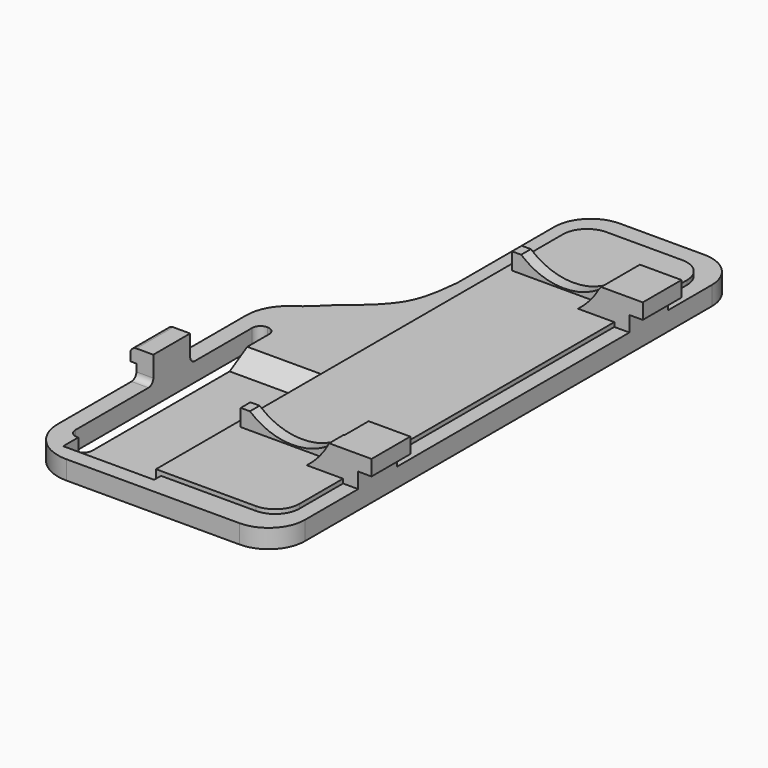
from build123d import *

# Parameters (mm, degrees)
F1_DEPTH     = 1.55
F3_DEPTH     = 0.35
F4_W         = 8.65
F4_H         = 1
F5_DEPTH     = 1.3
F7_W         = 4.25
F7_H         = 4
F8_DEPTH     = 2.55
F10_DEPTH    = 39.5010001
F11_W        = 4
F11_H        = 1.275
F12_DEPTH    = 1.1
F13_W        = 8.65
F13_H        = 1
F14_DEPTH    = 1.4
F15_DEPTH    = 38.0010001
F17_DEPTH    = 1.4
F18_T4_DEPTH = 11.4290603676
F19_T4_DEPTH = 10.6517870966
F20_W        = 1.4
F20_H        = 3.8
F21_DEPTH    = 2.2
F22_W        = 3.8
F22_H        = 1.1
F23_DEPTH    = 0.5
F24_R        = 0.5


# Not quite as in the source:
# - a fillet or chamfer that OpenCascade refuses, or shapes differently, is made with other operations: its cross-section is extruded or revolved along the edge and cut away or added


with BuildPart() as f1:
    # F0 (on Top) → F1 (new body)
    with BuildSketch(Plane.XY):
        with BuildLine():
            Line((-12.4797472133, -24.9172599055), (1.8202527867, -24.9172599055))
            ThreePointArc((1.8202527867, -24.9172599055), (3.9415731303, -24.038580249), (4.8202527867, -21.9172599055))
            Line((4.8202527867, -21.9172599055), (4.8202527867, 20.0827400945))
            ThreePointArc((4.8202527867, 20.0827400945), (3.9415731303, 22.2040604381), (1.8202527867, 23.0827400945))
            Line((1.8202527867, 23.0827400945), (-5.1797472133, 23.0827400945))
            ThreePointArc((-5.1797472133, 23.0827400945), (-7.3010675568, 22.2040604381), (-8.1797472133, 20.0827400945))
            Line((-8.1797472133, 20.0827400945), (-8.1797472133, 10.0827400945))
            add(Edge.make_bspline(
                [(-8.1797472133, 10.0827400945), (-8.4297074571, 7.300546721), (-9.1785947804, 5.6351239407), (-11.0454632546, 3.7753203501), (-12.7602456599, 2.4755173938), (-13.6481305175, 1.4367913649), (-14.42578763, 0.9165801451)],
                knots=[0, 0, 0, 0, 0.3064186573, 0.5153311453, 0.7233584291, 0.9057268673, 0.9057268673, 0.9057268673, 0.9057268673], degree=3))
            ThreePointArc((-14.42578763, 0.9165801451), (-15.5669094587, -0.3434616219), (-15.9797472133, -1.9925308353))
            Line((-15.9797472133, -1.9925308353), (-15.9797472133, -21.4172599055))
            ThreePointArc((-15.9797472133, -21.4172599055), (-14.9546209474, -23.8921336396), (-12.4797472133, -24.9172599055))
        make_face()
        with BuildLine():
            Line((-14.5797472133, -21.3672599055), (-14.5797472133, -3.1172599055))
            ThreePointArc((-14.5797472133, -3.1172599055), (-14.3747219601, -2.6222851587), (-13.8797472133, -2.4172599055))
            ThreePointArc((-13.8797472133, -2.4172599055), (-13.3847724664, -2.6222851587), (-13.1797472133, -3.1172599055))
            Line((-13.1797472133, -3.1172599055), (-13.1797472133, -21.3672599055))
            ThreePointArc((-13.1797472133, -21.3672599055), (-13.3847724664, -21.8622346523), (-13.8797472133, -22.0672599055))
            ThreePointArc((-13.8797472133, -22.0672599055), (-14.3747219601, -21.8622346523), (-14.5797472133, -21.3672599055))
        make_face(mode=Mode.SUBTRACT)
    extrude(amount=F1_DEPTH)

    # F2 (on face) → F3 (join)
    with BuildSketch(Plane.XY.offset(1.55)):
        with BuildLine():
            Line((1.5702527867, 21.0827400945), (-4.6797472133, 21.0827400945))
            ThreePointArc((-4.6797472133, 21.0827400945), (-6.0939607756, 20.4969536569), (-6.6797472133, 19.0827400945))
            Line((-6.6797472133, 19.0827400945), (-6.6797472133, -22.9172599055))
            Line((-6.6797472133, -22.9172599055), (1.5702527867, -22.9172599055))
            ThreePointArc((1.5702527867, -22.9172599055), (2.9844663491, -22.3314734679), (3.5702527867, -20.9172599055))
            Line((3.5702527867, -20.9172599055), (3.5702527867, 19.0827400945))
            ThreePointArc((3.5702527867, 19.0827400945), (2.9844663491, 20.4969536569), (1.5702527867, 21.0827400945))
        make_face()
    extrude(amount=F3_DEPTH)

    # F4 (on face) → F5 (join)
    with BuildSketch(Plane.XY.offset(1.9)):
        with Locations((-1.7547472133, 13.5827400945)):
            Rectangle(F4_W, F4_H)
        with Locations((-1.7547472133, -14.4172599055)):
            Rectangle(F4_W, F4_H)
    extrude(amount=F5_DEPTH)

    # F7 (on face) → F8 (join)
    with BuildSketch(Plane.XY.offset(1.55)):
        with Locations((2.6952527867, -14.4172599055)):
            Rectangle(F7_W, F7_H)
        with Locations((2.6952527867, 13.5827400945)):
            Rectangle(F7_W, F7_H)
    extrude(amount=F8_DEPTH)

    # F9 (on face) → F10 (cut, through all)
    with BuildSketch(Plane.XZ.offset(16.4172599055)):
        with BuildLine():
            Line((0.5702527867, 4.1), (0.5702527867, 1.9))
            ThreePointArc((0.5702527867, 1.9), (1.620780987, 2.8944421952), (2.4202527867, 4.1))
            Line((2.4202527867, 4.1), (0.5702527867, 4.1))
        make_face()
    extrude(amount=-F10_DEPTH, mode=Mode.SUBTRACT)

    # F11 (on face) → F12 (join)
    with BuildSketch(Plane.YZ.offset(4.8202527867)):
        with Locations((-14.4172599055, 3.4625)):
            Rectangle(F11_W, F11_H)
        with Locations((13.5827400945, 3.4625)):
            Rectangle(F11_W, F11_H)
    extrude(amount=F12_DEPTH)

    # F13 (on face) → F14 (join)
    with BuildSketch(Plane.XY.offset(1.9)):
        with Locations((-1.7547472133, -14.4172599055)):
            Rectangle(F13_W, F13_H)
        with Locations((-1.7547472133, 13.5827400945)):
            Rectangle(F13_W, F13_H)
    extrude(amount=F14_DEPTH)

    # F6 (on face) → F15 (cut, through all)
    with BuildSketch(Plane.XZ.offset(14.9172599055)):
        with BuildLine():
            Line((1.6002527867, 3.2), (-5.1997472133, 3.2))
            ThreePointArc((-5.1997472133, 3.2), (-1.7997472133, 2), (1.6002527867, 3.2))
        make_face()
        with BuildLine():
            ThreePointArc((3.6169194534, 7.4166666667), (-4.1367978237, 12.3032270339), (-5.1997472133, 3.2))
            Line((-5.1997472133, 3.2), (1.6002527867, 3.2))
            ThreePointArc((1.6002527867, 3.2), (3.0868131539, 5.0796160563), (3.6169194534, 7.4166666667))
        make_face()
    extrude(amount=-F15_DEPTH, mode=Mode.SUBTRACT)

    # F16 (on face) → F17 (cut)
    with BuildSketch(Plane.XY.offset(1.9)):
        Polygon((-6.6797472133, -22.9172599055), (-6.6797472133, -5.2834198549), (-13.1797472133, -5.2834198549), (-13.7797472133, -5.2834198549), (-13.7797472133, -23.7172599055), (-6.2646348961, -23.7172599055), (-6.2646348961, -22.9172599055), align=None)
    extrude(amount=-F17_DEPTH, mode=Mode.SUBTRACT)

    # F18: chamfer of 1.1 x 1.9052558883 on 1 edges, made by hand


with BuildPart() as f18_tool2:
    # F18_s3 → F18_t4 (new body)
    with BuildSketch(Plane.YZ.offset(-1.7506868456)):
        Polygon((-7.1886757432, 0.5), (-5.2834198549, 1.6), (-5.2834198549, 0.5), align=None)
    extrude(amount=-F18_T4_DEPTH)

    split(bisect_by=Plane.XY.offset(1.55), keep=Keep.BOTTOM)


with BuildPart() as f1_1:
    add(f1.part)

    # F18_t1: union F18_tool2
    add(f18_tool2.part)

    # F19: chamfer of 0.7 x 1.2124355653 on 1 edges, made by hand


with BuildPart() as f19_tool2:
    # F19_s3 → F19_t4 (new body)
    with BuildSketch(Plane.YZ.offset(-13.7797472133)):
        Polygon((-23.0172599055, 0.5), (-23.7172599055, 1.7124355653), (-23.7172599055, 0.5), align=None)
    extrude(amount=F19_T4_DEPTH)

    split(bisect_by=Plane.XY.offset(1.55), keep=Keep.BOTTOM)


with BuildPart() as f1_2:
    add(f1_1.part)

    # F19_t1: union F19_tool2
    add(f19_tool2.part)

    # F20 (on face) → F21 (join)
    with BuildSketch(Plane.XY.offset(1.55)):
        with Locations((-15.2797472133, -11.4172599055)):
            Rectangle(F20_W, F20_H)
    extrude(amount=F21_DEPTH)

    # F22 (on face) → F23 (join)
    with BuildSketch(Plane(origin=(-15.9797472133, 0, 0), x_dir=(0, -1, 0), z_dir=(-1, 0, 0))):
        with Locations((11.4172599055, 3.2)):
            Rectangle(F22_W, F22_H)
    extrude(amount=F23_DEPTH)

    # F24
    f24_edges = [f1_2.edges().sort_by_distance(p)[0] for p in [
        (-15.279747, -13.31726, 1.55),
        (-15.279747, -9.51726, 1.55),
        (-16.479747, -11.41726, 3.75),
    ]]
    fillet(f24_edges, radius=F24_R)


solid = f1_2.part
